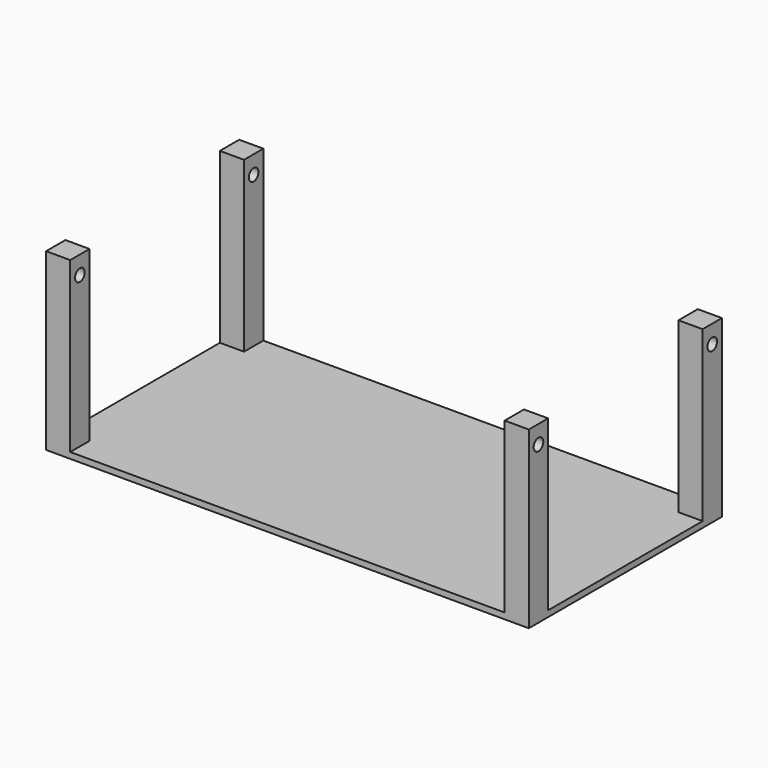
from build123d import *

# Parameters (mm, degrees)
F2_W             = 2000
F2_H             = 1000
F3_DEPTH         = 25
F4_W             = 100
F4_H             = 100
F5_DEPTH         = 700
F5_COPIES2_COUNT = 2
F6_R             = 25
F7_DEPTH         = 100
F7_COPIES2_COUNT = 2
F7_COPIES2_PITCH = 2102.379604


# Not quite as in the source:
# - a pattern or mirror of a feature is missing from the dataset's text; its kind, count and spacing are read off the source's solid


with BuildPart() as f3:
    # F2 (on Top) → F3 (new body)
    with BuildSketch(Plane.XY):
        Rectangle(F2_W, F2_H)
    extrude(amount=F3_DEPTH)

    # F4 (on face) → F5 (join)
    with BuildSketch(Plane.XY.offset(25)):
        with Locations((-950, 450)):
            Rectangle(F4_W, F4_H)
    f5 = extrude(amount=F5_DEPTH)

    # F5_copies: F5 across plane
    add(f5.mirror(Plane(origin=(0, 0, 0), x_dir=(0, 0, 1), z_dir=(1, 0, 0))))

    # F5_copies1: F5 across plane
    add(f5.mirror(Plane(origin=(0, 0, 0), x_dir=(0, 0, -1), z_dir=(0, -1, 0))))

    # F5_copies2: F5 ×2 about axis
    f5_copies2_axis = Axis((0, 0, 0), (0, 0, 1))
    for i in range(1, F5_COPIES2_COUNT):
        add(f5.rotate(f5_copies2_axis, i * 360 / F5_COPIES2_COUNT))

    # F6 (on face) → F7 (cut, through all)
    with BuildSketch(Plane.YZ.offset(-900)):
        with Locations((450, 650)):
            Circle(F6_R)
    f7 = extrude(amount=-F7_DEPTH, mode=Mode.SUBTRACT)

    # F7_copies: F7 across plane
    add(f7.mirror(Plane(origin=(0, 0, 0), x_dir=(0, 0, 1), z_dir=(1, 0, 0))), mode=Mode.SUBTRACT)

    # F7_copies1: F7 across plane
    add(f7.mirror(Plane(origin=(0, 0, 0), x_dir=(0, 0, -1), z_dir=(0, -1, 0))), mode=Mode.SUBTRACT)

    # F7_copies2: F7 ×2
    with Locations(*[Vector(0.9037378389, -0.4280863447, 0) * (i * F7_COPIES2_PITCH) for i in range(1, F7_COPIES2_COUNT)]):
        add(f7, mode=Mode.SUBTRACT)


solid = f3.part
